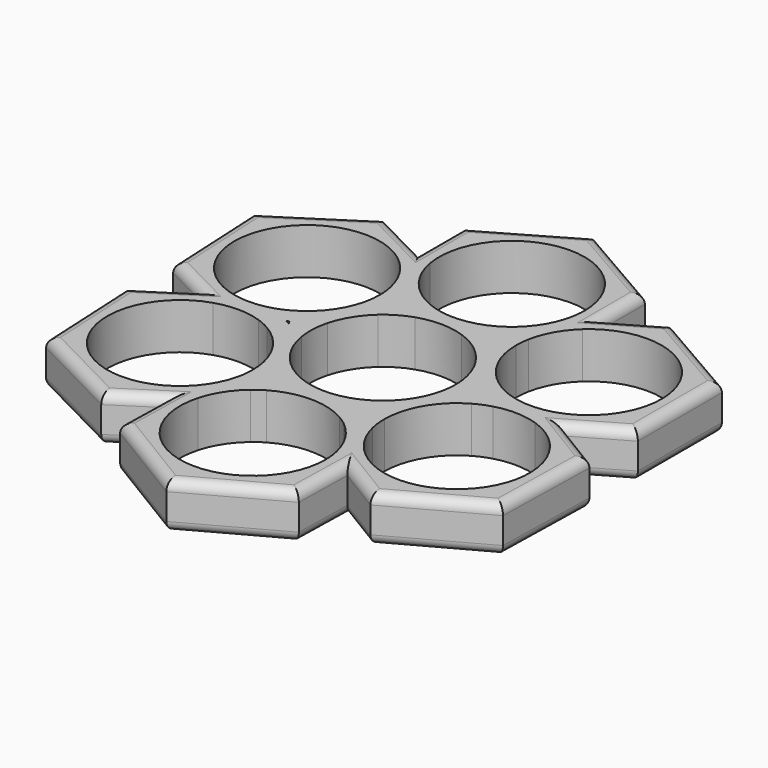
from build123d import *

# Parameters (mm, degrees)
F1_DEPTH = 7
F2_R     = 1.5


with BuildPart() as f1:
    # F0 (on Top) → F1 (new body)
    with BuildSketch(Plane.XY):
        with BuildLine():
            ThreePointArc((7.5985327445, 16.2733671096), (6.6383360142, 15.4839128008), (5.5957182097, 14.8070346876))
            Line((5.5957182097, 14.8070346876), (6.9770000586, 12.3927278963))
            Line((6.9770000586, 12.3927278963), (7.5985327445, 12.7515699599))
            Line((7.5985327445, 12.7515699599), (7.5985327445, 16.2733671096))
        make_face()
        with BuildLine():
            Line((6.9770000586, 12.3927278963), (5.5957182097, 14.8070346876))
            ThreePointArc((5.5957182097, 14.8070346876), (0.0524314036, 13.345033644), (-5.4791963127, 14.850547003))
            Line((-5.4791963127, 14.850547003), (-6.879406402, 12.4471684365))
            Line((-6.879406402, 12.4471684365), (-6.7752174647, 12.3870149255))
            Line((-6.7752174647, 12.3870149255), (6.9671049028, 12.3870149255))
            Line((6.9671049028, 12.3870149255), (6.9770000586, 12.3927278963))
        make_face()
        with BuildLine():
            Line((-6.879406402, 12.4471684365), (-5.4791963127, 14.850547003))
            ThreePointArc((-5.4791963127, 14.850547003), (-6.6962852306, 15.6723055756), (-7.7939497797, 16.6478695783))
            Line((-7.7939497797, 16.6478695783), (-7.6052014022, 12.8662063752))
            Line((-7.6052014022, 12.8662063752), (-6.879406402, 12.4471684365))
        make_face()
        Polygon((7.5985327445, 12.7515699599), (6.9770000586, 12.3927278963), (6.9802685839, 12.3870149255), (7.5985327445, 12.3870149255), align=None)
        Polygon((6.9802685839, 12.3870149255), (6.9770000586, 12.3927278963), (6.9671049028, 12.3870149255), align=None)
        with BuildLine():
            ThreePointArc((10.9729672137, 22.3352455746), (9.772675178, 19.0332522152), (7.5985327445, 16.2733671096))
            Line((7.5985327445, 16.2733671096), (7.5985327445, 12.7515699599))
            Line((7.5985327445, 12.7515699599), (10.5779157104, 14.4717175172))
            ThreePointArc((10.5779157104, 14.4717175172), (11.7782077461, 17.7737108767), (13.9523501796, 20.5335959823))
            Line((13.9523501796, 20.5335959823), (13.9523501796, 24.055393132))
            Line((13.9523501796, 24.055393132), (10.9729672137, 22.3352455746))
        make_face()
        Polygon((-6.7752174647, 12.3870149255), (-6.879406402, 12.4471684365), (-6.914451881, 12.3870149255), align=None)
        Polygon((-6.914451881, 12.3870149255), (-6.879406402, 12.4471684365), (-7.6052014022, 12.8662063752), (-7.5812842515, 12.3870149255), align=None)
        with BuildLine():
            Line((-7.6052014022, 12.8662063752), (-7.7939497797, 16.6478695783))
            ThreePointArc((-7.7939497797, 16.6478695783), (-9.7480287113, 19.3453218954), (-10.8116824399, 22.5017936946))
            Line((-10.8116824399, 22.5017936946), (-13.7604627415, 24.0135319721))
            Line((-13.7604627415, 24.0135319721), (-13.7604627415, 20.3526069909))
            ThreePointArc((-13.7604627415, 20.3526069909), (-11.7452424409, 17.7140604245), (-10.6026309913, 14.5967731554))
            Line((-10.6026309913, 14.5967731554), (-7.6052014022, 12.8662063752))
        make_face()
        Polygon((7.5985327445, 12.3870149255), (6.9802685839, 12.3870149255), (7.5985327445, 11.306367002), align=None)
        with BuildLine():
            Line((7.5985327445, 11.306367002), (6.9802685839, 12.3870149255))
            Line((6.9802685839, 12.3870149255), (6.9671049028, 12.3870149255))
            Line((6.9671049028, 12.3870149255), (3.6331063435, 10.4621299598))
            ThreePointArc((3.6331063435, 10.4621299598), (5.7431169216, 9.4695423873), (7.5985327445, 8.0571660732))
            Line((7.5985327445, 8.0571660732), (7.5985327445, 11.306367002))
        make_face()
        with BuildLine():
            Line((10.5779157104, 14.4717175172), (7.5985327445, 12.7515699599))
            Line((7.5985327445, 12.7515699599), (7.5985327445, 12.3870149255))
            Line((7.5985327445, 12.3870149255), (10.379939205, 12.3870149255))
            ThreePointArc((10.379939205, 12.3870149255), (10.4295444229, 13.4340559458), (10.5779157104, 14.4717175172))
        make_face()
        with BuildLine():
            Line((3.6331063435, 10.4621299598), (6.9671049028, 12.3870149255))
            Line((6.9671049028, 12.3870149255), (-6.7752174647, 12.3870149255))
            Line((-6.7752174647, 12.3870149255), (-3.5124473435, 10.5032537177))
            ThreePointArc((-3.5124473435, 10.5032537177), (0.0637372688, 11.0748165926), (3.6331063435, 10.4621299598))
        make_face()
        with BuildLine():
            ThreePointArc((11.170943719, 24.4199481664), (11.1213385012, 23.3729071461), (10.9729672137, 22.3352455746))
            Line((10.9729672137, 22.3352455746), (13.9523501796, 24.055393132))
            Line((13.9523501796, 24.055393132), (13.9523501796, 32.4199481664))
            Line((13.9523501796, 32.4199481664), (0.095943719, 40.4199481664))
            Line((0.095943719, 40.4199481664), (-13.7604627415, 32.4199481664))
            Line((-13.7604627415, 32.4199481664), (-13.7604627415, 24.0135319721))
            Line((-13.7604627415, 24.0135319721), (-10.8116824399, 22.5017936946))
            ThreePointArc((-10.8116824399, 22.5017936946), (-0.8667777594, 35.4530253598), (11.170943719, 24.4199481664))
        make_face()
        with BuildLine():
            Line((-6.7752174647, 12.3870149255), (-6.914451881, 12.3870149255))
            Line((-6.914451881, 12.3870149255), (-7.5286645779, 11.3327548239))
            Line((-7.5286645779, 11.3327548239), (-7.375394275, 8.2619116606))
            ThreePointArc((-7.375394275, 8.2619116606), (-5.5580731672, 9.5793239672), (-3.5124473435, 10.5032537177))
            Line((-3.5124473435, 10.5032537177), (-6.7752174647, 12.3870149255))
        make_face()
        Polygon((-7.5286645779, 11.3327548239), (-6.914451881, 12.3870149255), (-7.5812842515, 12.3870149255), align=None)
        with BuildLine():
            Line((-7.5812842515, 12.3870149255), (-7.6052014022, 12.8662063752))
            Line((-7.6052014022, 12.8662063752), (-10.6026309913, 14.5967731554))
            ThreePointArc((-10.6026309913, 14.5967731554), (-10.4357527907, 13.4974903942), (-10.379939205, 12.3870149255))
            Line((-10.379939205, 12.3870149255), (-7.5812842515, 12.3870149255))
        make_face()
        with BuildLine():
            Line((7.5985327445, 12.3870149255), (7.5985327445, 11.306367002))
            Line((7.5985327445, 11.306367002), (13.5098621825, 0.9741072832))
            Line((13.5098621825, 0.9741072832), (14.5267359748, 0.3870149255))
            Line((14.5267359748, 0.3870149255), (15.917439205, 2.7957835786))
            ThreePointArc((15.917439205, 2.7957835786), (11.8637078581, 6.8495149255), (10.379939205, 12.3870149255))
            Line((10.379939205, 12.3870149255), (7.5985327445, 12.3870149255))
        make_face()
        with BuildLine():
            Line((13.5098621825, 0.9741072832), (7.5985327445, 11.306367002))
            Line((7.5985327445, 11.306367002), (7.5985327445, 8.0571660732))
            ThreePointArc((7.5985327445, 8.0571660732), (9.5912313469, 5.5375), (10.7769768741, 2.5519393516))
            Line((10.7769768741, 2.5519393516), (13.5098621825, 0.9741072832))
        make_face()
        with BuildLine():
            Line((21.454939205, 28.3870149255), (13.9523501796, 24.055393132))
            Line((13.9523501796, 24.055393132), (13.9523501796, 20.5335959823))
            ThreePointArc((13.9523501796, 20.5335959823), (25.9026606185, 22.5296674005), (32.529939205, 12.3870149255))
            ThreePointArc((32.529939205, 12.3870149255), (30.3383270071, 5.7733135292), (24.6308789506, 1.7771595197))
            Line((24.6308789506, 1.7771595197), (27.6310759516, -0.0471908613))
            Line((27.6310759516, -0.0471908613), (35.3113456656, 4.3870149255))
            Line((35.3113456656, 4.3870149255), (35.3113456656, 20.3870149255))
            Line((35.3113456656, 20.3870149255), (21.454939205, 28.3870149255))
        make_face()
        with BuildLine():
            Line((-7.375394275, 8.2619116606), (-7.5286645779, 11.3327548239))
            Line((-7.5286645779, 11.3327548239), (-13.5501218282, 0.9972763088))
            Line((-13.5501218282, 0.9972763088), (-10.7062473349, 2.8340594568))
            ThreePointArc((-10.7062473349, 2.8340594568), (-9.439376871, 5.7925632743), (-7.375394275, 8.2619116606))
        make_face()
        with BuildLine():
            Line((-13.5501218282, 0.9972763088), (-7.5286645779, 11.3327548239))
            Line((-7.5286645779, 11.3327548239), (-7.5812842515, 12.3870149255))
            Line((-7.5812842515, 12.3870149255), (-10.379939205, 12.3870149255))
            ThreePointArc((-10.379939205, 12.3870149255), (-11.8637078581, 6.8495149255), (-15.917439205, 2.7957835786))
            Line((-15.917439205, 2.7957835786), (-14.5181117283, 0.3720772924))
            Line((-14.5181117283, 0.3720772924), (-13.5501218282, 0.9972763088))
        make_face()
        with BuildLine():
            Line((-13.7604627415, 20.3526069909), (-13.7604627415, 24.0135319721))
            Line((-13.7604627415, 24.0135319721), (-22.2525299156, 28.3671228431))
            Line((-22.2525299156, 28.3671228431), (-35.6929139722, 19.6863350671))
            Line((-35.6929139722, 19.6863350671), (-34.8953232616, 3.7062271495))
            Line((-34.8953232616, 3.7062271495), (-27.8297715403, 0.0839617055))
            Line((-27.8297715403, 0.0839617055), (-25.0171756289, 1.9005428466))
            ThreePointArc((-25.0171756289, 1.9005428466), (-30.9094894182, 18.1547792469), (-13.7604627415, 20.3526069909))
        make_face()
        Polygon((14.5267359748, 0.3870149255), (13.5098621825, 0.9741072832), (14.184695543, -0.2054164806), align=None)
        with BuildLine():
            Line((14.184695543, -0.2054164806), (13.5098621825, 0.9741072832))
            Line((13.5098621825, 0.9741072832), (10.7769768741, 2.5519393516))
            ThreePointArc((10.7769768741, 2.5519393516), (11.0002419037, 1.2846412182), (11.075, 0))
            ThreePointArc((11.075, 0), (11.0249592031, -1.0516175966), (10.8752890168, -2.093732027))
            Line((10.8752890168, -2.093732027), (14.1199666454, -0.31753022))
            Line((14.1199666454, -0.31753022), (14.184695543, -0.2054164806))
        make_face()
        with BuildLine():
            Line((-10.7062473349, 2.8340594568), (-13.5501218282, 0.9972763088))
            Line((-13.5501218282, 0.9972763088), (-14.2108644542, -0.1368496895))
            Line((-14.2108644542, -0.1368496895), (-10.924124391, -1.8218483172))
            ThreePointArc((-10.924124391, -1.8218483172), (-11.0628935884, 0.5176972578), (-10.7062473349, 2.8340594568))
        make_face()
        Polygon((-14.2108644542, -0.1368496895), (-13.5501218282, 0.9972763088), (-14.5181117283, 0.3720772924), (-14.2299239832, -0.1270785243), align=None)
        Polygon((14.5267359748, 0.3870149255), (14.184695543, -0.2054164806), (14.2181029544, -0.2638084302), (14.9551535767, 0.1396679077), align=None)
        Polygon((14.2181029544, -0.2638084302), (14.184695543, -0.2054164806), (14.1199666454, -0.31753022), align=None)
        with BuildLine():
            Line((15.917439205, 2.7957835786), (14.5267359748, 0.3870149255))
            Line((14.5267359748, 0.3870149255), (14.9551535767, 0.1396679077))
            Line((14.9551535767, 0.1396679077), (18.0667535, 1.8430203016))
            ThreePointArc((18.0667535, 1.8430203016), (16.9667429313, 2.2622078059), (15.917439205, 2.7957835786))
        make_face()
        with BuildLine():
            Line((-10.924124391, -1.8218483172), (-14.2108644542, -0.1368496895))
            Line((-14.2108644542, -0.1368496895), (-14.2176038945, -0.1484175438))
            Line((-14.2176038945, -0.1484175438), (-7.3245787425, -12.0874873249))
            Line((-7.3245787425, -12.0874873249), (-7.522177768, -8.1284971936))
            ThreePointArc((-7.522177768, -8.1284971936), (-9.7473058251, -5.257913479), (-10.924124391, -1.8218483172))
        make_face()
        Polygon((-14.2176038945, -0.1484175438), (-14.2108644542, -0.1368496895), (-14.2299239832, -0.1270785243), align=None)
        with BuildLine():
            Line((-14.8214349955, 0.1761688348), (-14.5181117283, 0.3720772924))
            Line((-14.5181117283, 0.3720772924), (-15.917439205, 2.7957835786))
            ThreePointArc((-15.917439205, 2.7957835786), (-16.9685211664, 2.2614197241), (-18.07045728, 1.8418308541))
            Line((-18.07045728, 1.8418308541), (-14.8214349955, 0.1761688348))
        make_face()
        with BuildLine():
            ThreePointArc((-18.07045728, 1.8418308541), (-21.5485390981, 1.3124104603), (-25.0171756289, 1.9005428466))
            Line((-25.0171756289, 1.9005428466), (-27.8297715403, 0.0839617055))
            Line((-27.8297715403, 0.0839617055), (-24.5807492558, -1.5817003138))
            ThreePointArc((-24.5807492558, -1.5817003138), (-21.1026674377, -1.05227992), (-17.6340309069, -1.6404123063))
            Line((-17.6340309069, -1.6404123063), (-14.8214349955, 0.1761688348))
            Line((-14.8214349955, 0.1761688348), (-18.07045728, 1.8418308541))
        make_face()
        with BuildLine():
            Line((14.9551535767, 0.1396679077), (14.2181029544, -0.2638084302))
            Line((14.2181029544, -0.2638084302), (15.600549121, -2.6801503024))
            ThreePointArc((15.600549121, -2.6801503024), (16.7937382754, -2.0896845497), (18.0491567586, -1.6466556623))
            Line((18.0491567586, -1.6466556623), (14.9551535767, 0.1396679077))
        make_face()
        with BuildLine():
            Line((15.600549121, -2.6801503024), (14.2181029544, -0.2638084302))
            Line((14.2181029544, -0.2638084302), (14.1199666454, -0.31753022))
            Line((14.1199666454, -0.31753022), (7.2417467081, -12.230956617))
            Line((7.2417467081, -12.230956617), (7.2415725605, -12.2386140294))
            Line((7.2415725605, -12.2386140294), (10.0254090893, -12.2495514658))
            ThreePointArc((10.0254090893, -12.2495514658), (11.5309224483, -6.7179237495), (15.600549121, -2.6801503024))
        make_face()
        with BuildLine():
            Line((7.2417467081, -12.230956617), (14.1199666454, -0.31753022))
            Line((14.1199666454, -0.31753022), (10.8752890168, -2.093732027))
            ThreePointArc((10.8752890168, -2.093732027), (9.6177729423, -5.4912720413), (7.3311180774, -8.3012247732))
            Line((7.3311180774, -8.3012247732), (7.2417467081, -12.230956617))
        make_face()
        with BuildLine():
            Line((18.0667535, 1.8430203016), (14.9551535767, 0.1396679077))
            Line((14.9551535767, 0.1396679077), (18.0491567586, -1.6466556623))
            ThreePointArc((18.0491567586, -1.6466556623), (21.3418152645, -1.2206969709), (24.6127709552, -1.7898100635))
            Line((24.6127709552, -1.7898100635), (27.6310759516, -0.0471908613))
            Line((27.6310759516, -0.0471908613), (24.6308789506, 1.7771595197))
            ThreePointArc((24.6308789506, 1.7771595197), (21.3438244109, 1.3125723435), (18.0667535, 1.8430203016))
        make_face()
        with BuildLine():
            Line((-7.3245787425, -12.0874873249), (-14.2176038945, -0.1484175438))
            Line((-14.2176038945, -0.1484175438), (-15.621127299, -2.5574832218))
            ThreePointArc((-15.621127299, -2.5574832218), (-11.5941763904, -6.6082364915), (-10.1212673307, -12.1268843852))
            ThreePointArc((-10.1212673307, -12.1268843852), (-10.1212887001, -12.1486405849), (-10.1213528083, -12.1703967006))
            Line((-10.1213528083, -12.1703967006), (-7.3198912537, -12.1814033841))
            Line((-7.3198912537, -12.1814033841), (-7.3245787425, -12.0874873249))
        make_face()
        with BuildLine():
            Line((-15.621127299, -2.5574832218), (-14.2176038945, -0.1484175438))
            Line((-14.2176038945, -0.1484175438), (-14.2299239832, -0.1270785243))
            Line((-14.2299239832, -0.1270785243), (-14.8214349955, 0.1761688348))
            Line((-14.8214349955, 0.1761688348), (-17.6340309069, -1.6404123063))
            ThreePointArc((-17.6340309069, -1.6404123063), (-16.6046263508, -2.0485681512), (-15.621127299, -2.5574832218))
        make_face()
        with BuildLine():
            Line((-24.5807492558, -1.5817003138), (-27.8297715403, 0.0839617055))
            Line((-27.8297715403, 0.0839617055), (-35.4342420979, -4.8275642436))
            Line((-35.4342420979, -4.8275642436), (-34.6366513873, -20.8076721612))
            Line((-34.6366513873, -20.8076721612), (-20.3986766201, -28.1069923028))
            Line((-20.3986766201, -28.1069923028), (-13.839442257, -23.870556704))
            Line((-13.839442257, -23.870556704), (-13.7589929816, -20.3331365904))
            ThreePointArc((-13.7589929816, -20.3331365904), (-30.7884710513, -17.662699843), (-24.5807492558, -1.5817003138))
        make_face()
        with BuildLine():
            Line((7.2373353106, -12.2385973816), (7.2417467081, -12.230956617))
            Line((7.2417467081, -12.230956617), (7.3311180774, -8.3012247732))
            ThreePointArc((7.3311180774, -8.3012247732), (5.4395783552, -9.6471038305), (3.3090313302, -10.5691029258))
            Line((3.3090313302, -10.5691029258), (6.0468714529, -12.2339201592))
            Line((6.0468714529, -12.2339201592), (7.2373353106, -12.2385973816))
        make_face()
        Polygon((7.2415725605, -12.2386140294), (7.2417467081, -12.230956617), (7.2373353106, -12.2385973816), align=None)
        with BuildLine():
            Line((35.1350399253, -4.6101777351), (27.6310759516, -0.0471908613))
            Line((27.6310759516, -0.0471908613), (24.6127709552, -1.7898100635))
            ThreePointArc((24.6127709552, -1.7898100635), (30.0879812412, -5.8217706079), (32.1753236117, -12.2930637812))
            ThreePointArc((32.1753236117, -12.2930637812), (25.7630492202, -22.3386904366), (13.9514653906, -20.7517546453))
            Line((13.9514653906, -20.7517546453), (13.874942038, -24.1165487356))
            Line((13.874942038, -24.1165487356), (20.7365399452, -28.2889276667))
            Line((20.7365399452, -28.2889276667), (34.7712562588, -20.6060416207))
            Line((34.7712562588, -20.6060416207), (35.1350399253, -4.6101777351))
        make_face()
        Polygon((-7.270243662, -12.1815984449), (-7.3245787425, -12.0874873249), (-7.3198912537, -12.1814033841), align=None)
        with BuildLine():
            Line((-7.522177768, -8.1284971936), (-7.3245787425, -12.0874873249))
            Line((-7.3245787425, -12.0874873249), (-7.270243662, -12.1815984449))
            Line((-7.270243662, -12.1815984449), (-5.863534628, -12.1871252747))
            Line((-5.863534628, -12.1871252747), (-3.0497633235, -10.646810258))
            ThreePointArc((-3.0497633235, -10.646810258), (-5.433871528, -9.650319436), (-7.522177768, -8.1284971936))
        make_face()
        with BuildLine():
            ThreePointArc((10.3204075038, -14.8325585553), (10.0968520288, -13.5497411959), (10.0254090893, -12.2495514658))
            Line((10.0254090893, -12.2495514658), (7.2415725605, -12.2386140294))
            Line((7.2415725605, -12.2386140294), (7.2253815737, -12.9505448966))
            Line((7.2253815737, -12.9505448966), (10.3204075038, -14.8325585553))
        make_face()
        Polygon((7.2253815737, -12.9505448966), (7.2415725605, -12.2386140294), (7.2373353106, -12.2385973816), (6.9299946835, -12.770926963), align=None)
        Polygon((6.9299946835, -12.770926963), (7.2373353106, -12.2385973816), (6.0468714529, -12.2339201592), align=None)
        with BuildLine():
            Line((-7.2808801797, -12.9630087423), (-7.3198912537, -12.1814033841))
            Line((-7.3198912537, -12.1814033841), (-10.1213528083, -12.1703967006))
            ThreePointArc((-10.1213528083, -12.1703967006), (-10.1987245034, -13.4344304689), (-10.419893146, -14.6813675876))
            Line((-10.419893146, -14.6813675876), (-7.2808801797, -12.9630087423))
        make_face()
        Polygon((-7.270243662, -12.1815984449), (-7.3198912537, -12.1814033841), (-7.2808801797, -12.9630087423), (-6.9299946835, -12.770926963), align=None)
        Polygon((-5.863534628, -12.1871252747), (-7.270243662, -12.1815984449), (-6.9299946835, -12.770926963), align=None)
        with BuildLine():
            ThreePointArc((3.3090313302, -10.5691029258), (0.1353313792, -11.0741731257), (-3.0497633235, -10.646810258))
            Line((-3.0497633235, -10.646810258), (-5.863534628, -12.1871252747))
            Line((-5.863534628, -12.1871252747), (6.0468714529, -12.2339201592))
            Line((6.0468714529, -12.2339201592), (3.3090313302, -10.5691029258))
        make_face()
        with BuildLine():
            ThreePointArc((-10.419893146, -14.6813675876), (-11.661076119, -17.7603339107), (-13.7589929816, -20.3331365904))
            Line((-13.7589929816, -20.3331365904), (-13.839442257, -23.870556704))
            Line((-13.839442257, -23.870556704), (-10.6757642468, -21.8272209419))
            ThreePointArc((-10.6757642468, -21.8272209419), (-9.3167414806, -18.7862127876), (-7.1149835804, -16.2868257383))
            Line((-7.1149835804, -16.2868257383), (-7.2808801797, -12.9630087423))
            Line((-7.2808801797, -12.9630087423), (-10.419893146, -14.6813675876))
        make_face()
        with BuildLine():
            ThreePointArc((13.9514653906, -20.7517546453), (11.6600133508, -18.084105758), (10.3204075038, -14.8325585553))
            Line((10.3204075038, -14.8325585553), (7.2253815737, -12.9505448966))
            Line((7.2253815737, -12.9505448966), (7.1488582211, -16.3153389869))
            ThreePointArc((7.1488582211, -16.3153389869), (9.4403102609, -18.9829878741), (10.7799161078, -22.2345350768))
            Line((10.7799161078, -22.2345350768), (13.874942038, -24.1165487356))
            Line((13.874942038, -24.1165487356), (13.9514653906, -20.7517546453))
        make_face()
        with BuildLine():
            Line((7.1488582211, -16.3153389869), (7.2253815737, -12.9505448966))
            Line((7.2253815737, -12.9505448966), (6.9299946835, -12.770926963))
            Line((6.9299946835, -12.770926963), (5.5375, -15.182798504))
            ThreePointArc((5.5375, -15.182798504), (6.3684050762, -15.7131776954), (7.1488582211, -16.3153389869))
        make_face()
        with BuildLine():
            Line((6.9299946835, -12.770926963), (6.0468714529, -12.2339201592))
            Line((6.0468714529, -12.2339201592), (-5.863534628, -12.1871252747))
            Line((-5.863534628, -12.1871252747), (-6.9299946835, -12.770926963))
            Line((-6.9299946835, -12.770926963), (-5.5375, -15.182798504))
            ThreePointArc((-5.5375, -15.182798504), (0, -13.699029851), (5.5375, -15.182798504))
            Line((5.5375, -15.182798504), (6.9299946835, -12.770926963))
        make_face()
        with BuildLine():
            Line((-6.9299946835, -12.770926963), (-7.2808801797, -12.9630087423))
            Line((-7.2808801797, -12.9630087423), (-7.1149835804, -16.2868257383))
            ThreePointArc((-7.1149835804, -16.2868257383), (-6.3502798538, -15.7004654588), (-5.5375, -15.182798504))
            Line((-5.5375, -15.182798504), (-6.9299946835, -12.770926963))
        make_face()
        with BuildLine():
            Line((-10.6757642468, -21.8272209419), (-13.839442257, -23.870556704))
            Line((-13.839442257, -23.870556704), (-14.0347163136, -32.456915897))
            Line((-14.0347163136, -32.456915897), (-0.3637836665, -40.7698937365))
            Line((-0.3637836665, -40.7698937365), (13.6709326471, -33.0870076904))
            Line((13.6709326471, -33.0870076904), (13.874942038, -24.1165487356))
            Line((13.874942038, -24.1165487356), (10.7799161078, -22.2345350768))
            ThreePointArc((10.7799161078, -22.2345350768), (11.0009816811, -23.4957391748), (11.075, -24.774029851))
            ThreePointArc((11.075, -24.774029851), (-1.486865153, -35.7487670695), (-10.6757642468, -21.8272209419))
        make_face()
    extrude(amount=F1_DEPTH)

    # F2
    f2_edges = [f1.edges().sort_by_distance(p)[0] for p in [
        (-31.362547, 1.895094, 0),
        (-31.632007, -2.371801, 0),
        (-35.035447, -12.817618, 0),
        (-27.517664, -24.457332, 0),
        (-17.119059, -25.988775, 0),
        (-13.937079, -28.163736, 0),
        (-7.19925, -36.613405, 0),
        (6.653574, -36.928451, 0),
        (13.772937, -28.601778, 0),
        (17.305741, -26.202738, 0),
        (27.753898, -24.447485, 0),
        (34.953148, -12.60811, 0),
        (31.383058, -2.328684, 0),
        (31.471211, 2.169912, 0),
        (35.311346, 12.387015, 0),
        (28.383142, 24.387015, 0),
        (17.703645, 26.221204, 0),
        (13.95235, 28.237671, 0),
        (7.024147, 36.419948, 0),
        (-6.83226, 36.419948, 0),
        (-13.760463, 28.21674, 0),
        (-18.006496, 26.190327, 0),
        (-28.972722, 24.026729, 0),
        (-35.294119, 11.696281, 0),
        (-28.972722, 24.026729, 7),
        (-35.294119, 11.696281, 7),
        (-31.362547, 1.895094, 7),
        (-31.632007, -2.371801, 7),
        (-35.035447, -12.817618, 7),
        (-27.517664, -24.457332, 7),
        (-17.119059, -25.988775, 7),
        (-13.937079, -28.163736, 7),
        (-7.19925, -36.613405, 7),
        (6.653574, -36.928451, 7),
        (13.772937, -28.601778, 7),
        (17.305741, -26.202738, 7),
        (27.753898, -24.447485, 7),
        (34.953148, -12.60811, 7),
        (31.383058, -2.328684, 7),
        (31.471211, 2.169912, 7),
        (35.311346, 12.387015, 7),
        (13.95235, 28.237671, 7),
        (7.024147, 36.419948, 7),
        (-6.83226, 36.419948, 7),
        (-13.760463, 28.21674, 7),
        (-18.006496, 26.190327, 7),
        (28.383142, 24.387015, 7),
        (17.703645, 26.221204, 7),
    ]]
    fillet(f2_edges, radius=F2_R)


solid = f1.part
